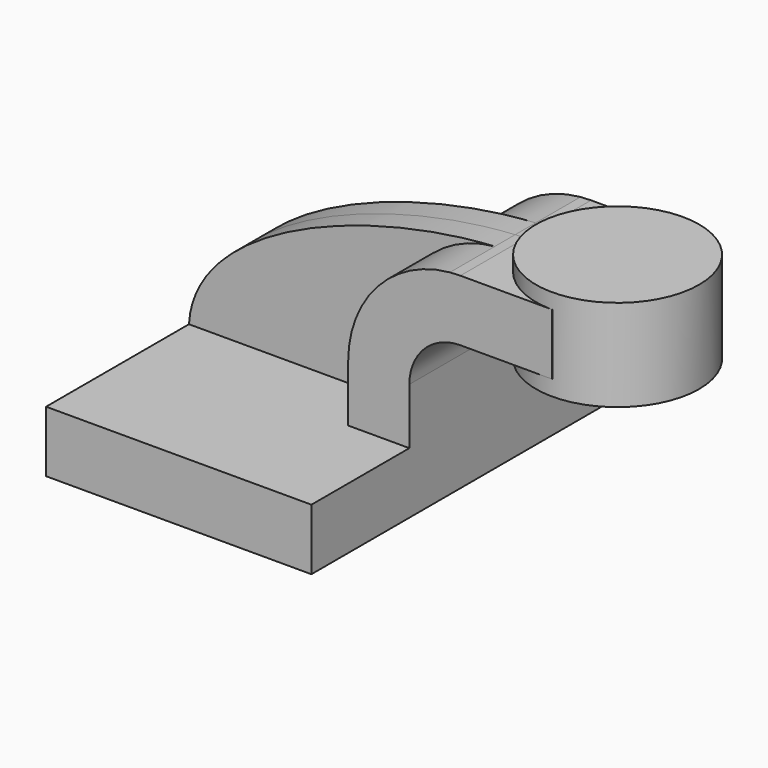
from build123d import *

# Parameters (mm, degrees)
F1_DEPTH = 63.5
F0_W     = 25.4
F0_H     = 19.05
F2_DEPTH = 25.4
F3_DEPTH = 7.9375


# Not quite as in the source:
# - a feature of the source that left no trace in its solid (it failed there, or was rolled back) is left out


with BuildPart() as f1:
    # F0 (on Front) → F1 (new body, symmetric)
    with BuildSketch(Plane.XZ):
        Polygon((22.225, 9.525), (-41.275, 9.525), (-41.275, -9.525), (41.275, -9.525), (41.275, 9.525), align=None)
    extrude(amount=F1_DEPTH, both=True)

    # F0 (on Front) → F2 (join, symmetric)
    with BuildSketch(Plane.XZ):
        with BuildLine():
            Line((22.225, 27.0002), (22.225, 9.525))
            Line((22.225, 9.525), (41.275, 9.525))
            Line((41.275, 9.525), (41.275, 27.0002))
            ThreePointArc((41.275, 27.0002), (45.9246798487, 38.2255201513), (57.15, 42.8752))
            Line((57.15, 42.8752), (60.325, 42.8752))
            Line((60.325, 42.8752), (60.325, 61.9252))
            Line((60.325, 61.9252), (57.15, 61.9252))
            add(Edge.make_bspline(
                [(53.8854342407, 61.7722898912), (54.9842067368, 61.8365871986), (56.0728453275, 61.8876096574), (57.15, 61.9252)],
                knots=[108.5245810491, 108.5245810491, 108.5245810491, 108.5245810491, 111.5045361635, 111.5045361635, 111.5045361635, 111.5045361635], degree=3))
            ThreePointArc((53.8854342407, 61.7722898912), (31.3258777096, 50.5133948686), (22.225, 27.0002))
        make_face()
        with Locations((73.025, 52.4002)):
            Rectangle(F0_W, F0_H)
    extrude(amount=F2_DEPTH, both=True)

    # F0 (on Front) → F3 (join, symmetric)
    with BuildSketch(Plane.XZ):
        with BuildLine():
            add(Edge.make_bspline(
                [(-41.275, 9.525), (-39.5856284224, 39.4828766469), (13.870125209, 59.4306981306), (53.8854342407, 61.7722898912)],
                knots=[0, 0, 0, 0, 108.5245810491, 108.5245810491, 108.5245810491, 108.5245810491], degree=3))
            Line((-41.275, 9.525), (22.225, 9.525))
            Line((22.225, 9.525), (22.225, 27.0002))
            ThreePointArc((22.225, 27.0002), (31.3258777096, 50.5133948686), (53.8854342407, 61.7722898912))
        make_face()
    extrude(amount=F3_DEPTH, both=True)


with BuildPart() as f4:
    # F0 (on Front) → F4 (revolve)
    with BuildSketch(Plane.XZ):
        Polygon((85.725, 66.675), (85.725, 61.9252), (85.725, 42.8752), (85.725, 38.1), (111.125, 38.1), (111.125, 66.675), align=None)
    revolve(axis=Axis((85.725, 0, 52.3875), (0, 0, 1)))


solid = Compound([f1.part, f4.part])
